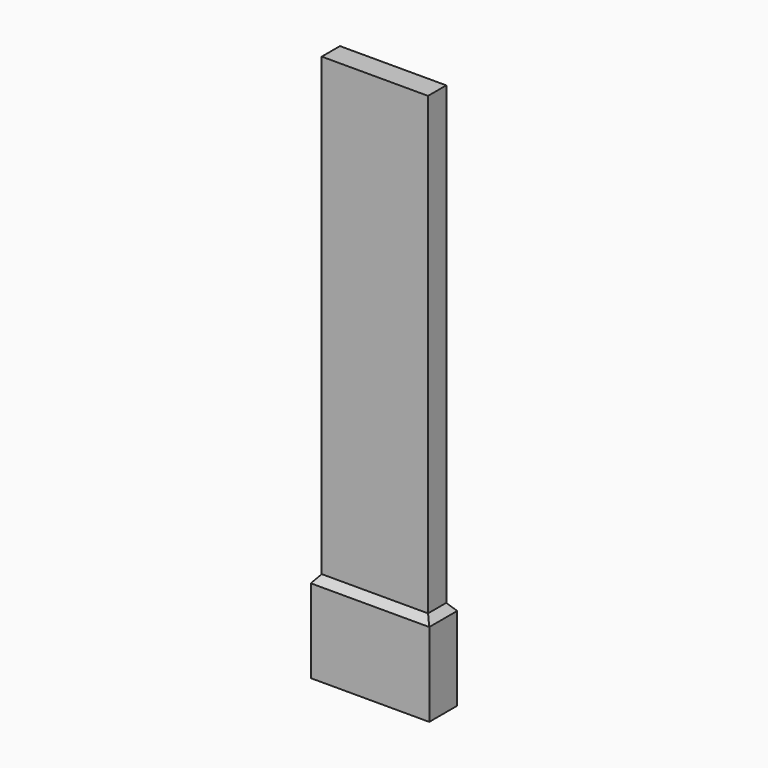
from build123d import *

# Parameters (mm, degrees)
F0_W     = 700
F0_H     = 150
F1_DEPTH = 3000
F0_W_2   = 780
F0_H_2   = 230
F2_DEPTH = 600
F3_SIZE2 = 39.99999
F3_SIZE  = 49.99999


# Not quite as in the source:
# - a fillet or chamfer is up to 0.001 mm smaller than in the source, because OpenCascade refuses the exact size


with BuildPart() as f1:
    # F0 (on Top) → F1 (new body)
    with BuildSketch(Plane.XY):
        Rectangle(F0_W, F0_H)
    extrude(amount=F1_DEPTH)


with BuildPart() as f2:
    # F0 (on Top) → F2 (new body)
    with BuildSketch(Plane.XY):
        Rectangle(F0_W_2, F0_H_2)
        Rectangle(F0_W, F0_H, mode=Mode.SUBTRACT)
    extrude(amount=-F2_DEPTH)

    # F3 (size 50 and 40 in the source; OpenCascade refuses exactly that, so slightly less here)
    f3_edges = [f2.edges().sort_by_distance(p)[0] for p in [
        (0, -115, 0),
        (390, 0, 0),
        (-390, 0, 0),
        (0, 115, 0),
    ]]
    chamfer(f3_edges, length=F3_SIZE, length2=F3_SIZE2)


solid = Compound([f1.part, f2.part])
